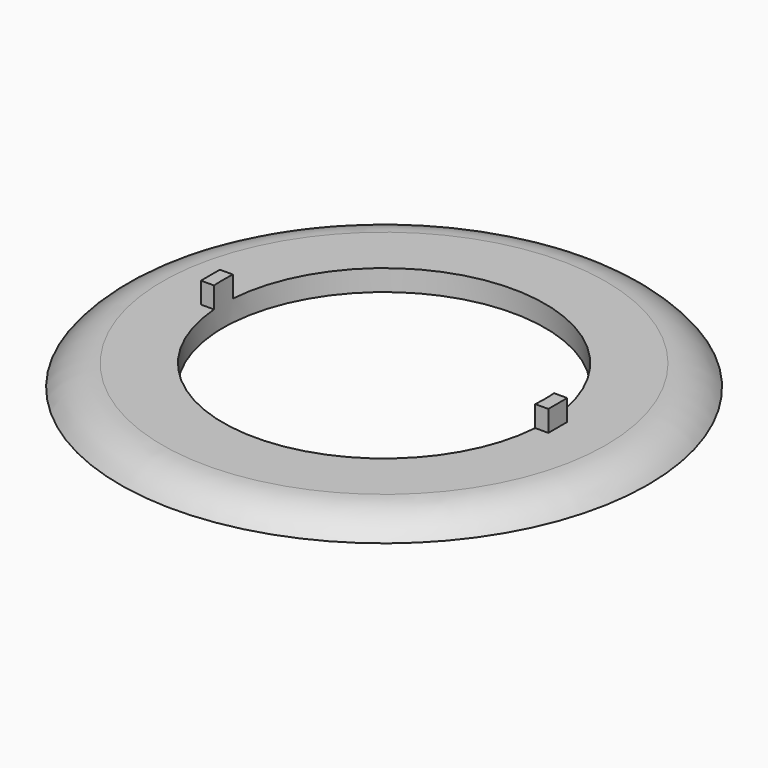
from build123d import *

# Parameters (mm, degrees)
F0_R     = 25
F1_DEPTH = 2
F3_DEPTH = 4


# Not quite as in the source:
# - a fillet or chamfer that OpenCascade refuses, or shapes differently, is made with other operations: its cross-section is extruded or revolved along the edge and cut away or added


with BuildPart() as f1:
    # F0 (on Top) → F1 (new body)
    with BuildSketch(Plane.XY):
        Circle(F0_R)
        with BuildLine():
            ThreePointArc((-15.2089073237, 1.1187662932), (0, 15.25), (15.2089073237, 1.1187662932))
            Line((15.2089073237, 1.1187662932), (16.45, 1.1187662932))
            Line((16.45, 1.1187662932), (16.45, -1.1187662932))
            Line((16.45, -1.1187662932), (15.2089073237, -1.1187662932))
            ThreePointArc((15.2089073237, -1.1187662932), (0, -15.25), (-15.2089073237, -1.1187662932))
            Line((-15.2089073237, -1.1187662932), (-16.45, -1.1187662932))
            Line((-16.45, -1.1187662932), (-16.45, 1.1187662932))
            Line((-16.45, 1.1187662932), (-15.2089073237, 1.1187662932))
        make_face(mode=Mode.SUBTRACT)
        with BuildLine():
            ThreePointArc((15.2089073237, 1.1187662932), (15.2397233683, 0.5597603565), (15.25, 0))
            ThreePointArc((15.25, 0), (15.2397233683, -0.5597603565), (15.2089073237, -1.1187662932))
            Line((15.2089073237, -1.1187662932), (16.45, -1.1187662932))
            Line((16.45, -1.1187662932), (16.45, 1.1187662932))
            Line((16.45, 1.1187662932), (15.2089073237, 1.1187662932))
        make_face()
        with BuildLine():
            ThreePointArc((-15.2089073237, -1.1187662932), (-15.25, 0), (-15.2089073237, 1.1187662932))
            Line((-15.2089073237, 1.1187662932), (-16.45, 1.1187662932))
            Line((-16.45, 1.1187662932), (-16.45, -1.1187662932))
            Line((-16.45, -1.1187662932), (-15.2089073237, -1.1187662932))
        make_face()
    extrude(amount=F1_DEPTH)

    # F2: fillet of radius 5 on 1 edges, made by hand

    # F2_s1 → F2_t2 (revolve, cut)
    with BuildSketch(Plane.XZ):
        with BuildLine():
            ThreePointArc((25, 0), (23.2360679775, 1.472135955), (21, 2))
            Line((21, 2), (25, 2))
            Line((25, 2), (25, 0))
        make_face()
    revolve(axis=Axis((0, 0, 2), (0, 0, 1)), mode=Mode.SUBTRACT)

    # F0 (on Top) → F3 (join)
    with BuildSketch(Plane.XY):
        with BuildLine():
            ThreePointArc((15.2089073237, 1.1187662932), (15.2397233683, 0.5597603565), (15.25, 0))
            ThreePointArc((15.25, 0), (15.2397233683, -0.5597603565), (15.2089073237, -1.1187662932))
            Line((15.2089073237, -1.1187662932), (16.45, -1.1187662932))
            Line((16.45, -1.1187662932), (16.45, 1.1187662932))
            Line((16.45, 1.1187662932), (15.2089073237, 1.1187662932))
        make_face()
        with BuildLine():
            ThreePointArc((-15.2089073237, -1.1187662932), (-15.25, 0), (-15.2089073237, 1.1187662932))
            Line((-15.2089073237, 1.1187662932), (-16.45, 1.1187662932))
            Line((-16.45, 1.1187662932), (-16.45, -1.1187662932))
            Line((-16.45, -1.1187662932), (-15.2089073237, -1.1187662932))
        make_face()
    extrude(amount=F3_DEPTH)


solid = f1.part
